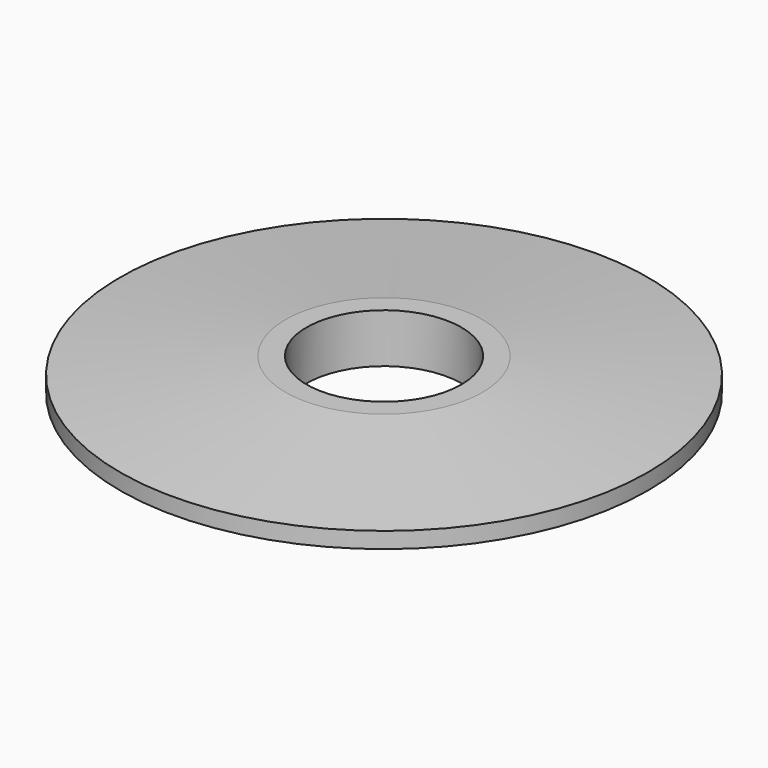
from build123d import *

# Parameters (mm, degrees)
F0_R     = 37.5
F0_R_2   = 11
F1_DEPTH = 3.5


# Not quite as in the source:
# - a pattern or mirror of a feature is missing from the dataset's text; its kind, count and spacing are read off the source's solid


with BuildPart() as f1:
    # F0 (on Top) → F1 (new body, symmetric)
    with BuildSketch(Plane.XY):
        Circle(F0_R)
        Circle(F0_R_2, mode=Mode.SUBTRACT)
    extrude(amount=F1_DEPTH, both=True)

    # F2 (on Right) → F3 (revolve, cut)
    with BuildSketch(Plane.YZ):
        Polygon((43.8578222282, 0.5), (43.8578222282, 0), (53.1842447817, 0), (53.1842447817, 16.8883297592), (14, 16.8883297592), (14, 3.5), align=None)
    f3 = revolve(axis=Axis((0, 0, 12.1004180983), (0, 0, 1)), mode=Mode.SUBTRACT)

    # F3_copies: F3 across plane
    add(f3.mirror(Plane(origin=(0, 0, 0), x_dir=(-1, 0, 0), z_dir=(0, 0, -1))), mode=Mode.SUBTRACT)


solid = f1.part
